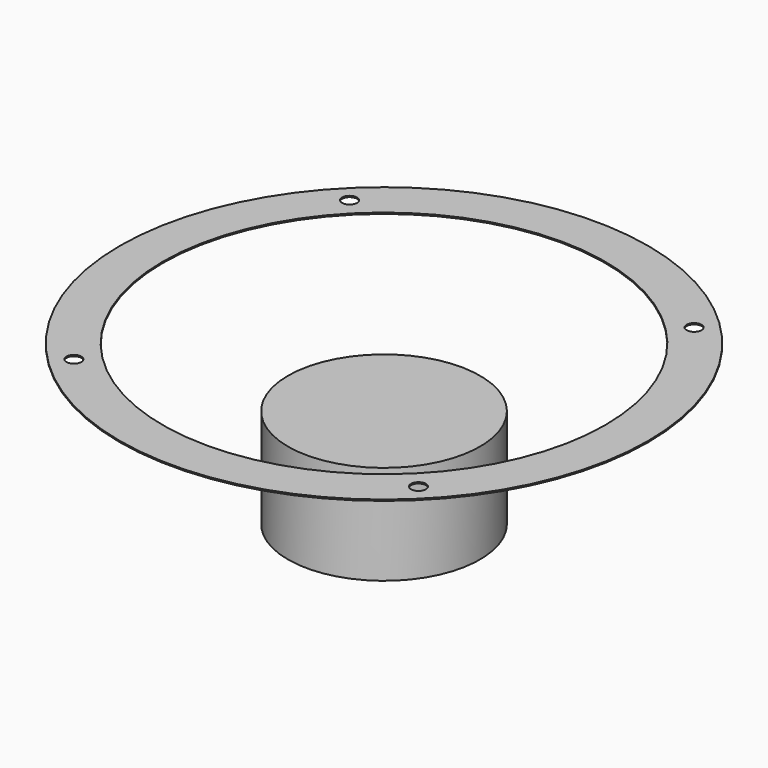
from build123d import *

# Parameters (mm, degrees)
F0_W = 8.6182065606
F0_H = 0.2540749386
F6_D = 3


# Not quite as in the source:
# - a feature names something its author has since deleted; it is built from what else it names
# - the program builds the solid bodies; features that only make, move or delete a surface that nothing else refers to are left out


with BuildPart() as f3:
    # F0 (on Front) → F3 (revolve)
    with BuildSketch(Plane.XZ):
        Polygon((-16.4538044245, 0), (-19.3070657551, 0), (-19.3070657551, -20), (0, -20), (0, 0), align=None)
    revolve(axis=Axis((0, 0, 10.1666413248), (0, 0, -1)))


with BuildPart() as f3b:
    # F0 (on Front) → F3, piece 2 (revolve)
    with BuildSketch(Plane.XZ):
        with Locations((-48.8091032803, 11.8729625307)):
            Rectangle(F0_W, F0_H)
    revolve(axis=Axis((0, 0, 10.1666413248), (0, 0, -1)))

    # F6 (through all)
    with Locations(Plane.XY.offset(12)):
        with Locations((-34.6482322781, 34.6482322781), (34.6482322781, 34.6482322781), (34.6482322781, -34.6482322781), (-34.6482322781, -34.6482322781)):
            Hole(F6_D / 2)


solid = Compound([f3.part, f3b.part])
